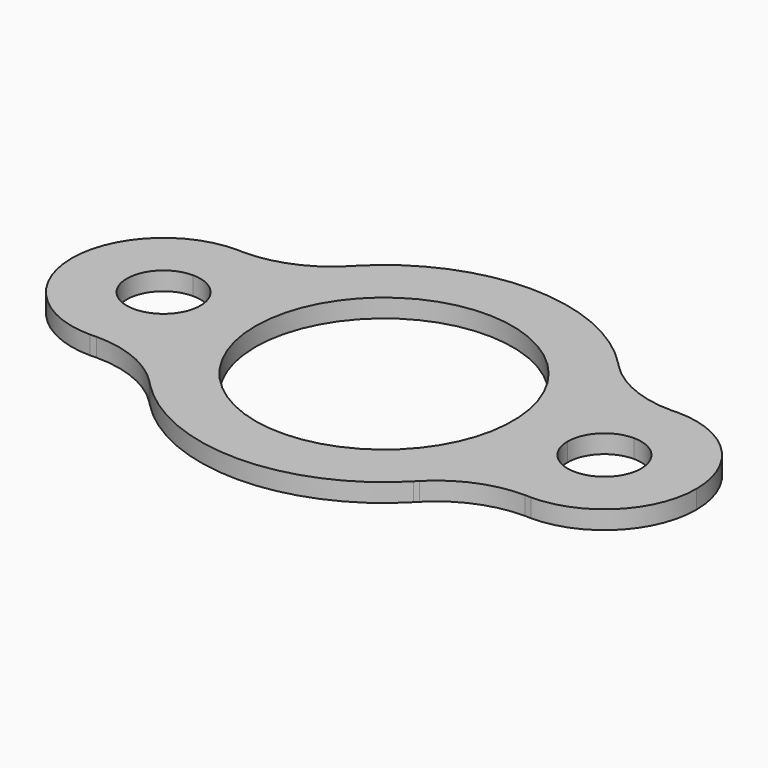
from build123d import *

# Parameters (mm, degrees)
F1_DEPTH = 6.35


with BuildPart() as f1:
    # F0 (on Top) → F1 (new body)
    with BuildSketch(Plane.XY):
        with BuildLine():
            ThreePointArc((57.94375, -25.976370723), (48.024670033, -14.636026826), (44.45, 0))
            ThreePointArc((44.45, 0), (0, -44.45), (-44.45, 0))
            ThreePointArc((-44.45, 0), (-48.024670033, -14.636026826), (-57.94375, -25.976370723))
            ThreePointArc((-57.94375, -25.976370723), (-53.0122296555, -34.9564515783), (-46.7007710297, -43.0265962543))
            ThreePointArc((-46.7007710297, -43.0265962543), (-46.1408199964, -43.6066686624), (-45.5932687094, -44.1984597966))
            ThreePointArc((-45.5932687094, -44.1984597966), (0, -63.5), (45.5932687094, -44.1984597966))
            ThreePointArc((45.5932687094, -44.1984597966), (46.1408199964, -43.6066686624), (46.7007710297, -43.0265962543))
            ThreePointArc((46.7007710297, -43.0265962543), (53.0122296555, -34.9564515783), (57.94375, -25.976370723))
        make_face()
        with BuildLine():
            ThreePointArc((57.94375, 25.976370723), (48.024670033, 14.636026826), (44.45, 0))
            Line((44.45, 0), (63.5, 0))
            ThreePointArc((63.5, 0), (62.0954029096, 13.2819779212), (57.94375, 25.976370723))
        make_face()
        with BuildLine():
            ThreePointArc((-44.45, 0), (0, 44.45), (44.45, 0))
            ThreePointArc((44.45, 0), (48.024670033, 14.636026826), (57.94375, 25.976370723))
            ThreePointArc((57.94375, 25.976370723), (53.0122296555, 34.9564515783), (46.7007710297, 43.0265962543))
            ThreePointArc((46.7007710297, 43.0265962543), (46.1408199964, 43.6066686624), (45.5932687094, 44.1984597966))
            ThreePointArc((45.5932687094, 44.1984597966), (0, 63.5), (-45.5932687094, 44.1984597966))
            ThreePointArc((-45.5932687094, 44.1984597966), (-46.1408199964, 43.6066686624), (-46.7007710297, 43.0265962543))
            ThreePointArc((-46.7007710297, 43.0265962543), (-53.0122296555, 34.9564515783), (-57.94375, 25.976370723))
            ThreePointArc((-57.94375, 25.976370723), (-48.024670033, 14.636026826), (-44.45, 0))
        make_face()
        with BuildLine():
            Line((63.5, 0), (44.45, 0))
            ThreePointArc((44.45, 0), (48.024670033, -14.636026826), (57.94375, -25.976370723))
            ThreePointArc((57.94375, -25.976370723), (62.0954029096, -13.2819779212), (63.5, 0))
        make_face()
        with BuildLine():
            ThreePointArc((-57.94375, -25.976370723), (-48.024670033, -14.636026826), (-44.45, 0))
            Line((-44.45, 0), (-63.5, 0))
            ThreePointArc((-63.5, 0), (-62.0954029096, -13.2819779212), (-57.94375, -25.976370723))
        make_face()
        with BuildLine():
            Line((-63.5, 0), (-44.45, 0))
            ThreePointArc((-44.45, 0), (-48.024670033, 14.636026826), (-57.94375, 25.976370723))
            ThreePointArc((-57.94375, 25.976370723), (-62.0954029096, 13.2819779212), (-63.5, 0))
        make_face()
        with BuildLine():
            ThreePointArc((76.2, -12.7), (67.2197438789, -8.9802561211), (63.5, 0))
            ThreePointArc((63.5, 0), (62.0954029096, -13.2819779212), (57.94375, -25.976370723))
            ThreePointArc((57.94375, -25.976370723), (65.6047024614, -29.9299543947), (74.0468101417, -31.6769044168))
            ThreePointArc((74.0468101417, -31.6769044168), (75.1239218386, -31.6982296864), (76.2, -31.75))
            Line((76.2, -31.75), (76.2, -12.7))
        make_face()
        with BuildLine():
            ThreePointArc((57.94375, 25.976370723), (62.0954029096, 13.2819779212), (63.5, 0))
            ThreePointArc((63.5, 0), (67.2197438789, 8.9802561211), (76.2, 12.7))
            Line((76.2, 12.7), (76.2, 31.75))
            ThreePointArc((76.2, 31.75), (75.1239218386, 31.6982296864), (74.0468101417, 31.6769044168))
            ThreePointArc((74.0468101417, 31.6769044168), (65.6047024614, 29.9299543947), (57.94375, 25.976370723))
        make_face()
        with BuildLine():
            ThreePointArc((46.7007710297, 43.0265962543), (53.0122296555, 34.9564515783), (57.94375, 25.976370723))
            ThreePointArc((57.94375, 25.976370723), (65.6047024614, 29.9299543947), (74.0468101417, 31.6769044168))
            ThreePointArc((74.0468101417, 31.6769044168), (59.2262146143, 34.5867715285), (46.7007710297, 43.0265962543))
        make_face()
        with BuildLine():
            ThreePointArc((74.0468101417, -31.6769044168), (65.6047024614, -29.9299543947), (57.94375, -25.976370723))
            ThreePointArc((57.94375, -25.976370723), (53.0122296555, -34.9564515783), (46.7007710297, -43.0265962543))
            ThreePointArc((46.7007710297, -43.0265962543), (59.2262146143, -34.5867715285), (74.0468101417, -31.6769044168))
        make_face()
        with BuildLine():
            ThreePointArc((-76.2, 12.7), (-67.2197438789, 8.9802561211), (-63.5, 0))
            ThreePointArc((-63.5, 0), (-62.0954029096, 13.2819779212), (-57.94375, 25.976370723))
            ThreePointArc((-57.94375, 25.976370723), (-65.6047024614, 29.9299543947), (-74.0468101417, 31.6769044168))
            ThreePointArc((-74.0468101417, 31.6769044168), (-75.1239218386, 31.6982296864), (-76.2, 31.75))
            Line((-76.2, 31.75), (-76.2, 12.7))
        make_face()
        with BuildLine():
            ThreePointArc((-57.94375, -25.976370723), (-62.0954029096, -13.2819779212), (-63.5, 0))
            ThreePointArc((-63.5, 0), (-67.2197438789, -8.9802561211), (-76.2, -12.7))
            Line((-76.2, -12.7), (-76.2, -31.75))
            ThreePointArc((-76.2, -31.75), (-75.1239218386, -31.6982296864), (-74.0468101417, -31.6769044168))
            ThreePointArc((-74.0468101417, -31.6769044168), (-65.6047024614, -29.9299543947), (-57.94375, -25.976370723))
        make_face()
        with BuildLine():
            ThreePointArc((-74.0468101417, 31.6769044168), (-65.6047024614, 29.9299543947), (-57.94375, 25.976370723))
            ThreePointArc((-57.94375, 25.976370723), (-53.0122296555, 34.9564515783), (-46.7007710297, 43.0265962543))
            ThreePointArc((-46.7007710297, 43.0265962543), (-59.2262146143, 34.5867715285), (-74.0468101417, 31.6769044168))
        make_face()
        with BuildLine():
            ThreePointArc((-46.7007710297, -43.0265962543), (-53.0122296555, -34.9564515783), (-57.94375, -25.976370723))
            ThreePointArc((-57.94375, -25.976370723), (-65.6047024614, -29.9299543947), (-74.0468101417, -31.6769044168))
            ThreePointArc((-74.0468101417, -31.6769044168), (-59.2262146143, -34.5867715285), (-46.7007710297, -43.0265962543))
        make_face()
        with BuildLine():
            Line((76.2, 31.75), (76.2, 12.7))
            ThreePointArc((76.2, 12.7), (85.1802561211, 8.9802561211), (88.9, 0))
            ThreePointArc((88.9, 0), (85.1802561211, -8.9802561211), (76.2, -12.7))
            Line((76.2, -12.7), (76.2, -31.75))
            ThreePointArc((76.2, -31.75), (98.6506403027, -22.4506403027), (107.95, 0))
            ThreePointArc((107.95, 0), (98.6506403027, 22.4506403027), (76.2, 31.75))
        make_face()
        with BuildLine():
            ThreePointArc((-76.2, -12.7), (-88.9, 0), (-76.2, 12.7))
            Line((-76.2, 12.7), (-76.2, 31.75))
            ThreePointArc((-76.2, 31.75), (-107.95, 0), (-76.2, -31.75))
            Line((-76.2, -31.75), (-76.2, -12.7))
        make_face()
    extrude(amount=F1_DEPTH)


solid = f1.part
